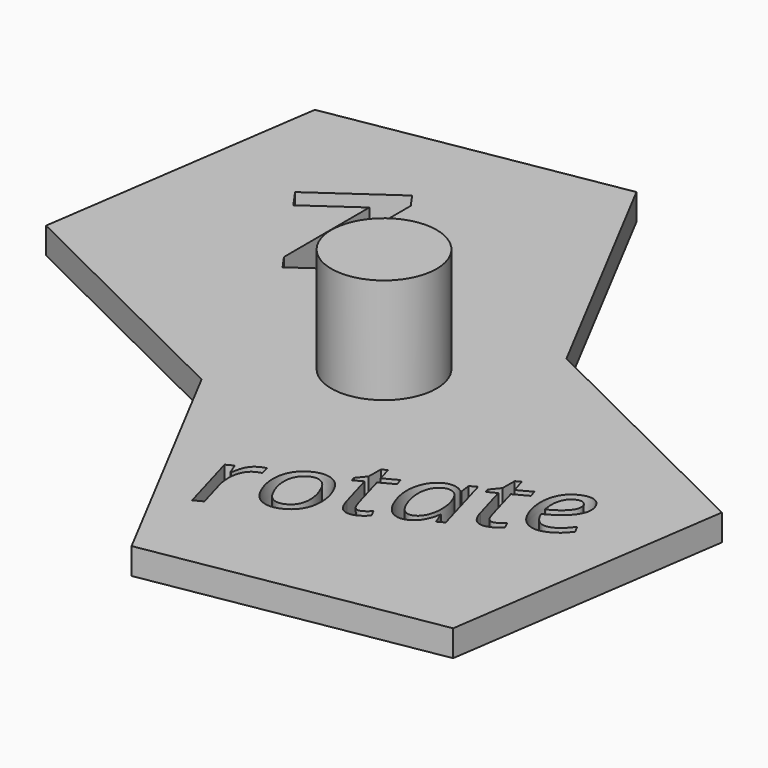
from build123d import *

# Parameters (mm, degrees)
F2_DEPTH       = 5.08
F3_DEPTH       = 5.08
F4_R           = 10.16
F5_DEPTH       = 25.4
F5_DEPTH_BACK  = 25.4
F6_TEXT_SIZE   = 34.4603632887
F7_DEPTH       = 5.08
F7_DEPTH_BACK  = 25.4
F8_TEXT_SIZE   = 23.0636758109
F9_DEPTH       = 25.4
F10_DEPTH      = 25.4
F10_DEPTH_BACK = 25.4


# Not quite as in the source:
# - Text() gives the source's letters only with a copy of the font that has no kerning and outlines rounded to 1/6400 em; it was checked with that copy


with BuildPart() as f2:
    # F1 (on Top) → F2 (new body)
    with BuildSketch(Plane.XY):
        Polygon((19.3392245842, 19.8052295832), (-19.3392245842, -19.8052295832), (6.3802626104, -68.8309257425), (60.9542290383, -59.5200131246), (68.963307997, -4.7398565011), align=None)
    extrude(amount=F2_DEPTH)

    # F0 (on Top) → F3 (join)
    with BuildSketch(Plane.XY):
        Polygon((-19.3392245842, -19.8052295832), (19.3392245842, 19.8052295832), (-6.3802626104, 68.8309257425), (-60.9542290383, 59.5200131246), (-68.963307997, 4.7398565011), align=None)
    extrude(amount=F3_DEPTH)

    # F6 (on Top) → F7 (cut, two sides)
    with BuildSketch(Plane.XY) as f7_sk:
        with Locations(Location((-33.3372028404, 15.8965714602), (0, 0, 35))):
            Text('Z', F6_TEXT_SIZE, font='Open Sans', font_style=FontStyle.BOLD, text_align=(TextAlign.LEFT, TextAlign.BOTTOM))
    extrude(amount=-F7_DEPTH, mode=Mode.SUBTRACT)
    extrude(f7_sk.sketch, amount=F7_DEPTH_BACK, mode=Mode.SUBTRACT)

    # F8 (on Top) → F9 (cut)
    with BuildSketch(Plane.XY):
        with Locations(Location((3.5913520494, -51.8003206674), (0, 0, 27.9384442473))):
            Text('rotate', F8_TEXT_SIZE, font='Open Sans', font_style=FontStyle.ITALIC, text_align=(TextAlign.LEFT, TextAlign.BOTTOM))
    extrude(amount=-F9_DEPTH, mode=Mode.SUBTRACT)

    # F8 (on Top) → F10 (cut, two sides)
    with BuildSketch(Plane.XY) as f10_sk:
        with Locations(Location((3.5913520494, -51.8003206674), (0, 0, 27.9384442473))):
            Text('rotate', F8_TEXT_SIZE, font='Open Sans', font_style=FontStyle.ITALIC, text_align=(TextAlign.LEFT, TextAlign.BOTTOM))
    extrude(amount=-F10_DEPTH, mode=Mode.SUBTRACT)
    extrude(f10_sk.sketch, amount=F10_DEPTH_BACK, mode=Mode.SUBTRACT)


with BuildPart() as f5:
    # F4 (on Top) → F5 (new body, two sides)
    with BuildSketch(Plane.XY) as f5_sk:
        Circle(F4_R)
    extrude(amount=-F5_DEPTH)
    extrude(f5_sk.sketch, amount=F5_DEPTH_BACK)


solid = Compound([f2.part, f5.part])
